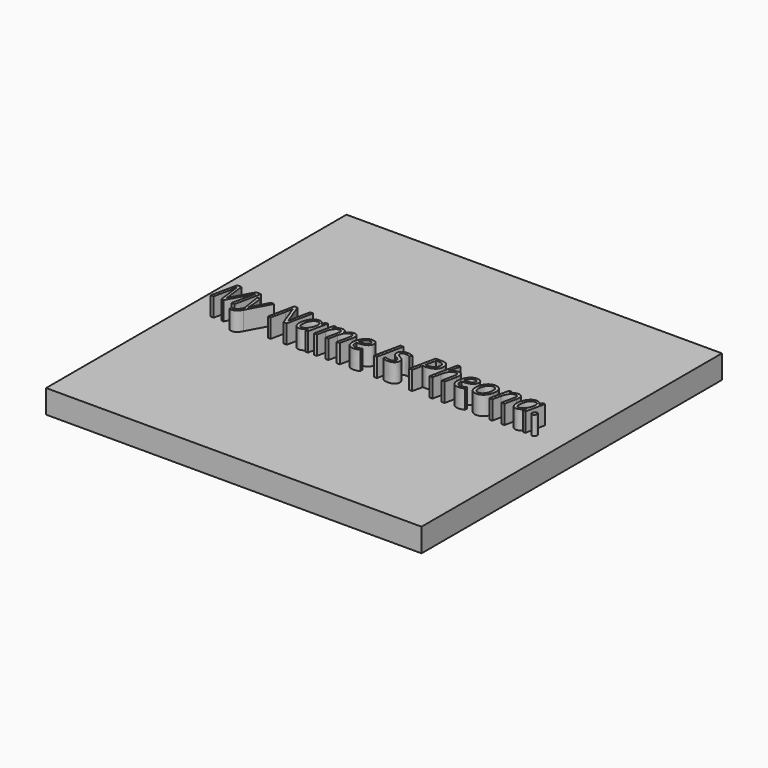
from build123d import *

# Parameters (mm, degrees)
F0_W         = 101.6
F0_H         = 101.6
F1_DEPTH     = 6.35
F2_TEXT_SIZE = 9.9237786266
F3_DEPTH     = 5.08


# Not quite as in the source:
# - Text() gives the source's letters only with a copy of the font that has no kerning and outlines rounded to 1/6400 em; it was checked with that copy


with BuildPart() as f1:
    # F0 (on Top) → F1 (new body)
    with BuildSketch(Plane.XY):
        Rectangle(F0_W, F0_H)
    extrude(amount=F1_DEPTH)

    # F2 (on face) → F3 (join)
    with BuildSketch(Plane.XY.offset(6.35)):
        with Locations((-44.45, -3.5725603056)):
            Text('My Name Is Pheona.', F2_TEXT_SIZE, font='Open Sans', font_style=FontStyle.ITALIC, text_align=(TextAlign.LEFT, TextAlign.BOTTOM))
    extrude(amount=F3_DEPTH)


solid = f1.part
